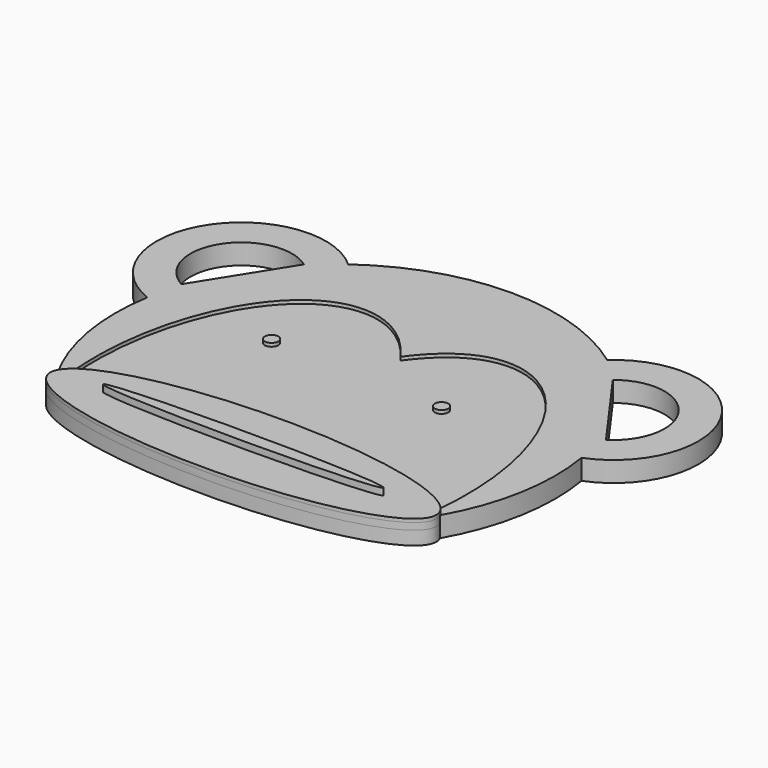
from build123d import *

# Parameters (mm, degrees)
F1_DEPTH = 1
F2_DEPTH = 1.5
F3_R     = 1
F4_DEPTH = 0.5
F6_DEPTH = 25
F8_DEPTH = 1
F9_DEPTH = 2


with BuildPart() as f1:
    # F0 (on Top) → F1 (new body)
    with BuildSketch(Plane.XY):
        with BuildLine():
            ThreePointArc((-19.1235008121, 26.278160451), (-38.1324321193, 23.5727762192), (-32.0550449903, 5.359486045))
            ThreePointArc((-32.0550449903, 5.359486045), (-32.0021823164, -5.6665974787), (-28.2657794627, -16.0404398744))
            add(Edge.make_bspline(
                [(28.2657794627, -16.0404398744), (25.0596180916, -9.5), (0, -9.5), (-25.0596180916, -9.5), (-28.2657794627, -16.0404398744)],
                knots=[0.1282929916, 0.1282929916, 0.1282929916, 1.5707963268, 1.5707963268, 3.013299662, 3.013299662, 3.013299662], degree=2, weights=[1, 0.75097981, 1, 0.75097981, 1]))
            ThreePointArc((28.2657794627, -16.0404398744), (32.0021823164, -5.6665974787), (32.0550449903, 5.359486045))
            ThreePointArc((32.0550449903, 5.359486045), (38.1324321193, 23.5727762192), (19.1235008121, 26.278160451))
            ThreePointArc((19.1235008121, 26.278160451), (0, 32.5), (-19.1235008121, 26.278160451))
        make_face()
        with BuildLine():
            add(Edge.make_bspline(
                [(28.2657794627, -16.0404398744), (25.0596180916, -9.5), (0, -9.5), (-25.0596180916, -9.5), (-28.2657794627, -16.0404398744)],
                knots=[0.1282929916, 0.1282929916, 0.1282929916, 1.5707963268, 1.5707963268, 3.013299662, 3.013299662, 3.013299662], degree=2, weights=[1, 0.75097981, 1, 0.75097981, 1]))
            add(Edge.make_bspline(
                [(-28.2657794627, -16.0404398744), (-32.1538432676, -23.9719332087), (-1.8269216338, -24.4845748919), (28.5, -24.9972165751), (28.5, -17)],
                knots=[3.013299662, 3.013299662, 3.013299662, 4.6482424846, 4.6482424846, 6.2831853072, 6.2831853072, 6.2831853072], degree=2, weights=[1, 0.6840677914, 1, 0.6840677914, 1]))
            add(Edge.make_bspline(
                [(28.5, -17), (28.5, -16.518240323), (28.2657794627, -16.0404398744)],
                knots=[0, 0, 0, 0.1282929916, 0.1282929916, 0.1282929916], degree=2, weights=[1, 0.9979433189, 1]))
        make_face()
    extrude(amount=F1_DEPTH)

    # F0 (on Top) → F2 (join)
    with BuildSketch(Plane.XY):
        with BuildLine():
            add(Edge.make_bspline(
                [(28.2657794627, -16.0404398744), (25.0596180916, -9.5), (0, -9.5), (-25.0596180916, -9.5), (-28.2657794627, -16.0404398744)],
                knots=[0.1282929916, 0.1282929916, 0.1282929916, 1.5707963268, 1.5707963268, 3.013299662, 3.013299662, 3.013299662], degree=2, weights=[1, 0.75097981, 1, 0.75097981, 1]))
            add(Edge.make_bspline(
                [(-28.2657794627, -16.0404398744), (-32.1538432676, -23.9719332087), (-1.8269216338, -24.4845748919), (28.5, -24.9972165751), (28.5, -17)],
                knots=[3.013299662, 3.013299662, 3.013299662, 4.6482424846, 4.6482424846, 6.2831853072, 6.2831853072, 6.2831853072], degree=2, weights=[1, 0.6840677914, 1, 0.6840677914, 1]))
            add(Edge.make_bspline(
                [(28.5, -17), (28.5, -16.518240323), (28.2657794627, -16.0404398744)],
                knots=[0, 0, 0, 0.1282929916, 0.1282929916, 0.1282929916], degree=2, weights=[1, 0.9979433189, 1]))
        make_face()
    extrude(amount=F2_DEPTH)

    # F3 (on face) → F4 (cut)
    with BuildSketch(Plane.XY.offset(1)):
        with BuildLine():
            add(Edge.make_bspline(
                [(27.2298485398, -14.785946603), (34.6781532449, 61.4301931961), (0, 12)],
                knots=[4.5465331149, 4.5465331149, 4.5465331149, 6.9772320681, 6.9772320681, 6.9772320681], degree=2, weights=[1, 0.348009318, 1]))
            add(Edge.make_bspline(
                [(0, 12), (-34.6781532449, 61.4301931961), (-27.2298485398, -14.785946603)],
                knots=[5.5891385462, 5.5891385462, 5.5891385462, 8.0198374994, 8.0198374994, 8.0198374994], degree=2, weights=[1, 0.348009318, 1]))
            add(Edge.make_bspline(
                [(-27.2298485438, -14.7859465983), (-27.1235005909, -14.6953694452), (-27.0148324256, -14.6074553179), (-26.9041242662, -14.5220377708), (-26.7916116729, -14.4389689728), (-26.6774911689, -14.3581129382), (-26.5619238942, -14.2793410628), (-26.4450372953, -14.2025299637), (-26.1154259475, -13.9933190312), (-25.9001007444, -13.8650502344), (-25.6815764788, -13.7421154762), (-25.4603422242, -13.6240265652), (-25.2367872003, -13.5103782123), (-25.0112167389, -13.4008190797), (-24.7838582265, -13.2950409799), (-24.1815269893, -13.0260138383), (-23.8039763572, -12.8686274032), (-23.4229953928, -12.7194286319), (-23.0391676676, -12.5775726359), (-22.6529452943, -12.442384814), (-22.2646725462, -12.3132991432), (-21.8745928745, -12.1898396478), (-21.0075231865, -11.9280985148), (-20.5298402909, -11.7923034154), (-20.0501673244, -11.6634792789), (-19.5687883822, -11.5410606749), (-19.0859317536, -11.4245881786), (-18.6017794799, -11.3136725414), (-18.1164723782, -11.2079754108), (-16.5759163532, -10.8887891981), (-15.5169354155, -10.6935580552), (-14.4542494004, -10.5185387591), (-13.3886584475, -10.3618210579), (-12.3207818781, -10.2219317761), (-11.2510694701, -10.0977602294), (-10.1798249497, -9.9884221743), (-7.9905872411, -9.7941373106), (-6.872614176, -9.7103865584), (-5.7535809166, -9.6412114374), (-4.6337472088, -9.586067236), (-3.5133459581, -9.5445749391), (-2.3925855443, -9.5164852067), (-1.2716508776, -9.5016647144), (-0.0658567051, -9.4999867866), (0.0188272492, -9.4999449156), (0.103506139, -9.4999785093), (0.1882859732, -9.5000876991), (0.273221364, -9.500273079), (0.358315594, -9.5005353037), (0.4435206851, -9.5008746872), (1.9146357736, -9.5080581365), (3.300394752, -9.5351034815), (4.6857535149, -9.5824945952), (6.0703729366, -9.6505743409), (7.4538305978, -9.7399869052), (8.8356188507, -9.8516936697), (10.215135598, -9.987094422), (12.2470780769, -10.2251595717), (12.9017942823, -10.3078129902), (13.5557282033, -10.3965638624), (14.2087777108, -10.491687712), (14.8608158428, -10.5935051159), (15.5116886245, -10.7023952032), (16.1612112004, -10.8188191074), (17.3779682579, -11.0526761832), (17.9455245563, -11.1682417081), (18.5117085891, -11.2904454713), (19.0763384267, -11.419745162), (19.6391657791, -11.5566868167), (20.1998710662, -11.7019244141), (20.7580501445, -11.8562724484), (21.6401455013, -12.1177532327), (21.9660283027, -12.2182108793), (22.2907322232, -12.322429107), (22.6141230493, -12.430665212), (22.9360300506, -12.5432111617), (23.2562413481, -12.6604065516), (23.5744953864, -12.7826620273), (24.1535181548, -13.0169134178), (24.4149432173, -13.1271804164), (24.6745873797, -13.2416031142), (24.9322211673, -13.3605257562), (25.187532615, -13.4843455592), (25.4401209542, -13.613525357), (25.6894788059, -13.748629127), (26.1059183514, -13.9891577643), (26.2747150273, -14.0909802774), (26.4413094594, -14.1962143234), (26.6055249122, -14.3052048432), (26.7670432139, -14.418298237), (26.9253904774, -14.5358566012), (27.0799325858, -14.6582621601), (27.2298485569, -14.7859465829)],
                knots=[0.0277398129, 0.0277398129, 0.0277398129, 0.0277398129, 0.0277398129, 0.0277398129, 0.0277398129, 0.0277398129, 0.0277398129, 0.046627634, 0.046627634, 0.046627634, 0.046627634, 0.046627634, 0.046627634, 0.046627634, 0.080449246, 0.080449246, 0.080449246, 0.080449246, 0.080449246, 0.080449246, 0.080449246, 0.1355918365, 0.1355918365, 0.1355918365, 0.1355918365, 0.1355918365, 0.1355918365, 0.1355918365, 0.202503631, 0.202503631, 0.202503631, 0.202503631, 0.202503631, 0.202503631, 0.202503631, 0.3475356161, 0.3475356161, 0.3475356161, 0.3475356161, 0.3475356161, 0.3475356161, 0.3475356161, 0.4985180369, 0.4985180369, 0.4985180369, 0.4985180369, 0.4985180369, 0.4985180369, 0.4985180369, 0.5099461608, 0.5099461608, 0.5099461608, 0.5099461608, 0.5099461608, 0.5099461608, 0.5099461608, 0.695804126, 0.695804126, 0.695804126, 0.695804126, 0.695804126, 0.695804126, 0.695804126, 0.7842990266, 0.7842990266, 0.7842990266, 0.7842990266, 0.7842990266, 0.7842990266, 0.7842990266, 0.8619845652, 0.8619845652, 0.8619845652, 0.8619845652, 0.8619845652, 0.8619845652, 0.8619845652, 0.9077400087, 0.9077400087, 0.9077400087, 0.9077400087, 0.9077400087, 0.9077400087, 0.9077400087, 0.9458317068, 0.9458317068, 0.9458317068, 0.9458317068, 0.9458317068, 0.9458317068, 0.9458317068, 0.972362644, 0.972362644, 0.972362644, 0.972362644, 0.972362644, 0.972362644, 0.972362644, 0.972362644, 0.972362644], degree=8))
        make_face()
        with Locations((-14.3968807533, 6.2048500404)):
            Circle(F3_R, mode=Mode.SUBTRACT)
        with Locations((11.3892154768, 5.359486045)):
            Circle(F3_R, mode=Mode.SUBTRACT)
    extrude(amount=-F4_DEPTH, mode=Mode.SUBTRACT)

    # F5 (on face) → F6 (cut)
    with BuildSketch(Plane.XY.offset(1)):
        with BuildLine():
            Line((-31.0509426966, 10.3938811723), (-23.101764943, 23.074992048))
            ThreePointArc((-23.101764943, 23.074992048), (-33.8546927027, 20.9834508474), (-31.0509426966, 10.3938811723))
        make_face()
        with BuildLine():
            ThreePointArc((31.4558537042, 10.6280912224), (33.5940096319, 21.3718470474), (22.7316116782, 22.788995838))
            Line((22.7316116782, 22.788995838), (31.4558537042, 10.6280912224))
        make_face()
    extrude(amount=-F6_DEPTH, mode=Mode.SUBTRACT)

    # F7 (on face) → F8 (join)
    with BuildSketch(Plane.XY.offset(1.5)):
        with BuildLine():
            add(Edge.make_bspline(
                [(-20.6742249429, -17), (-20.6742249429, -18.7320508076), (10.3371124715, -17.8660254038), (41.3484498858, -17), (10.3371124715, -16.1339745962), (-20.6742249429, -15.2679491924), (-20.6742249429, -17)],
                knots=[0, 0, 0, 2.0943951024, 2.0943951024, 4.1887902048, 4.1887902048, 6.2831853072, 6.2831853072, 6.2831853072], degree=2, weights=[1, 0.5, 1, 0.5, 1, 0.5, 1]))
        make_face()
    extrude(amount=F8_DEPTH)

    # F9 (add): a face of the model
    f9_faces = [f1.faces().sort_by_distance(p)[0] for p in [
        (0.0027966544, 4.1583376267, 0),
    ]]
    extrude(f9_faces, amount=F9_DEPTH)


solid = f1.part
